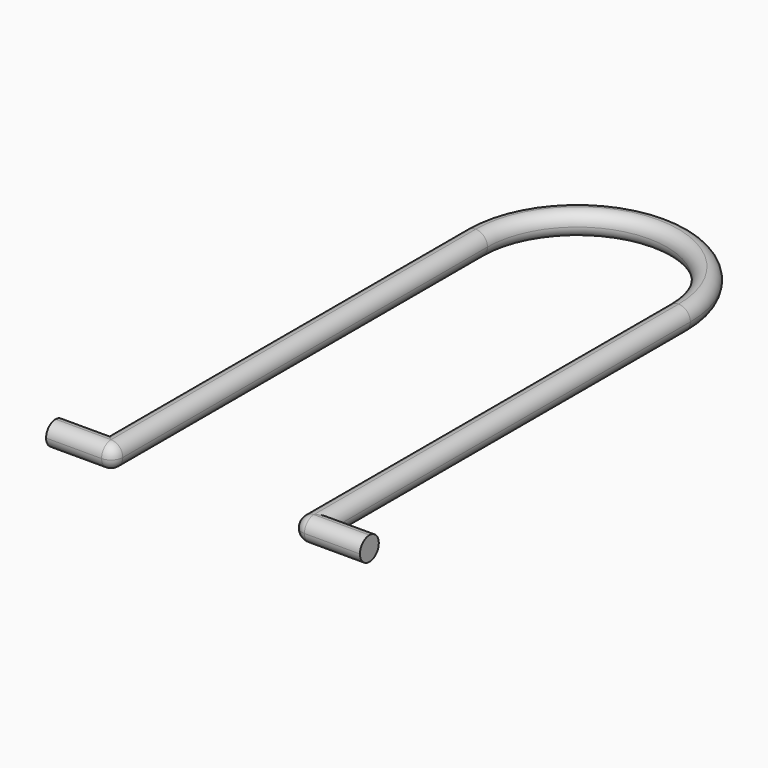
from build123d import *

# Parameters (mm, degrees)
F1_DEPTH = 1.3462
F2_R     = 0.67309


# Not quite as in the source:
# - a fillet or chamfer is up to 0.001 mm smaller than in the source, because OpenCascade refuses the exact size


with BuildPart() as f1:
    # F0 (on Top) → F1 (new body)
    with BuildSketch(Plane.XY):
        with BuildLine():
            Line((-3.8481, 0), (0, 0))
            Line((0, 0), (0, 26.7462))
            ThreePointArc((0, 26.7462), (5.1277647, 31.8739647), (10.2555294, 26.7462))
            Line((10.2555294, 26.7462), (10.2555294, 0))
            Line((10.2555294, 0), (14.1036294, 0))
            Line((14.1036294, 0), (14.1036294, 1.3462))
            Line((14.1036294, 1.3462), (11.6017294, 1.3462))
            Line((11.6017294, 1.3462), (11.6017294, 26.7462))
            ThreePointArc((11.6017294, 26.7462), (5.1277647, 33.2201647), (-1.3462, 26.7462))
            Line((-1.3462, 26.7462), (-1.3462, 1.3462))
            Line((-1.3462, 1.3462), (-3.8481, 1.3462))
            Line((-3.8481, 1.3462), (-3.8481, 0))
        make_face()
    extrude(amount=F1_DEPTH)

    # F2 (radius 0.6731 in the source; OpenCascade refuses exactly that, so slightly less here)
    f2_edges = [f1.edges().sort_by_distance(p)[0] for p in [
        (0, 0, 0.6731),
        (-1.92405, 0, 1.3462),
        (-1.92405, 0, 0),
        (0, 13.3731, 1.3462),
        (0, 13.3731, 0),
        (5.127765, 31.873965, 1.3462),
        (5.127765, 31.873965, 0),
        (10.255529, 13.3731, 1.3462),
        (11.601729, 14.0462, 1.3462),
        (11.601729, 14.0462, 0),
        (5.127765, 33.220165, 0),
        (5.127765, 33.220165, 1.3462),
        (10.255529, 0, 0.6731),
        (10.255529, 13.3731, 0),
        (12.179579, 0, 1.3462),
        (12.179579, 0, 0),
        (12.852679, 1.3462, 0),
        (12.852679, 1.3462, 1.3462),
        (-2.59715, 1.3462, 1.3462),
        (-2.59715, 1.3462, 0),
    ]]
    fillet(f2_edges, radius=F2_R)


solid = f1.part
